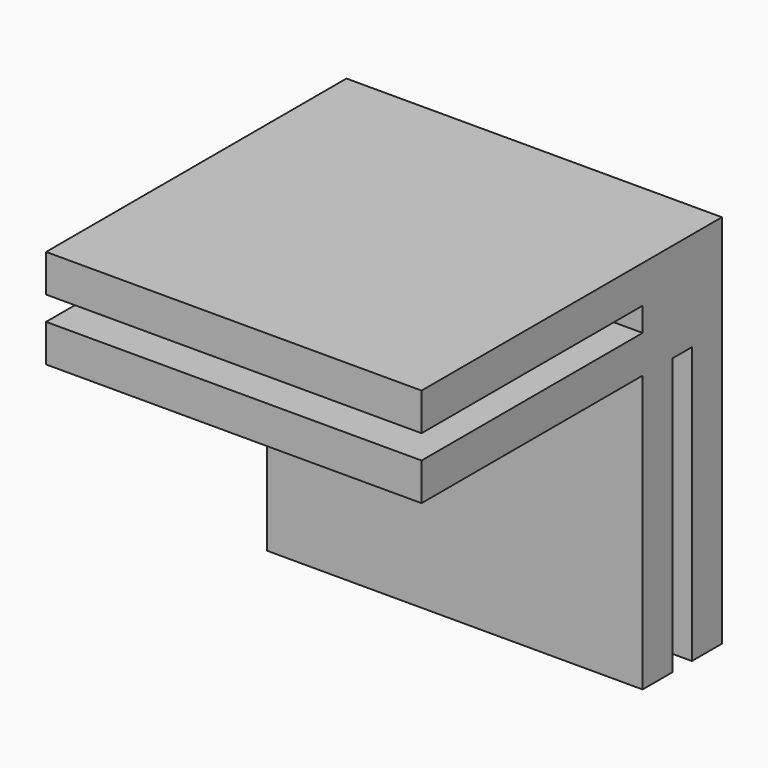
from build123d import *

# Parameters (mm, degrees)
F0_W     = 50
F0_H     = 50
F1_DEPTH = 5
F2_W     = 5
F2_H     = 50
F3_DEPTH = 50
F4_W     = 50
F4_H     = 5
F5_DEPTH = 36.8
F6_W     = 3.2
F6_H     = 8.2
F7_DEPTH = 50


# Not quite as in the source:
# - a feature names something its author has since deleted; it is built from what else it names


with BuildPart() as f1:
    # F0 (on Top) → F1 (new body)
    with BuildSketch(Plane.XY):
        Rectangle(F0_W, F0_H)
    extrude(amount=F1_DEPTH)

    # F2 (on face) → F3 (join, through all)
    with BuildSketch(Plane(origin=(-25, 0, 0), x_dir=(0, -1, 0), z_dir=(-1, 0, 0))):
        with Locations((-22.5, -20)):
            Rectangle(F2_W, F2_H)
        with Locations((-14.3, -20)):
            Rectangle(F2_W, F2_H)
    extrude(amount=-F3_DEPTH)

    # F4 (on face) → F5 (join, through all)
    with BuildSketch(Plane.XZ.offset(-11.8)):
        with Locations((0, -5.7)):
            Rectangle(F4_W, F4_H)
    extrude(amount=F5_DEPTH)

    # F6 (on face) → F7 (join, through all)
    with BuildSketch(Plane(origin=(-25, 0, 0), x_dir=(0, -1, 0), z_dir=(-1, 0, 0))):
        with Locations((-18.4, -4.1)):
            Rectangle(F6_W, F6_H)
    extrude(amount=-F7_DEPTH)


solid = f1.part
